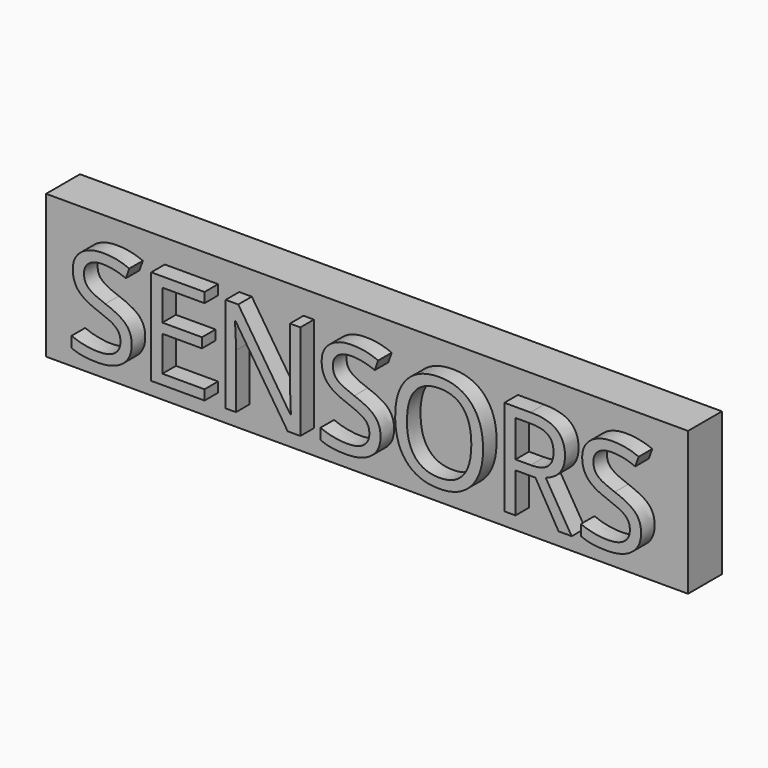
from build123d import *

# Parameters (mm, degrees)
F0_W         = 757.4373483658
F0_H         = 169.1906601191
F1_DEPTH     = 50
F2_TEXT_SIZE = 157.9731237143
F3_DEPTH     = 70


# Not quite as in the source:
# - Text() gives the source's letters only with a copy of the font that has no kerning and outlines rounded to 1/6400 em; it was checked with that copy


with BuildPart() as f1:
    # F0 (on Front) → F1 (new body)
    with BuildSketch(Plane.XZ):
        with Locations((378.7186741829, 84.5953300595)):
            Rectangle(F0_W, F0_H)
    extrude(amount=F1_DEPTH)

    # F2 (on Front) → F3 (join)
    with BuildSketch(Plane.XZ):
        with Locations((37.8743372858, 28.5236276686)):
            Text('SENSORS', F2_TEXT_SIZE, font='Open Sans', text_align=(TextAlign.LEFT, TextAlign.BOTTOM))
    extrude(amount=F3_DEPTH)


solid = f1.part
